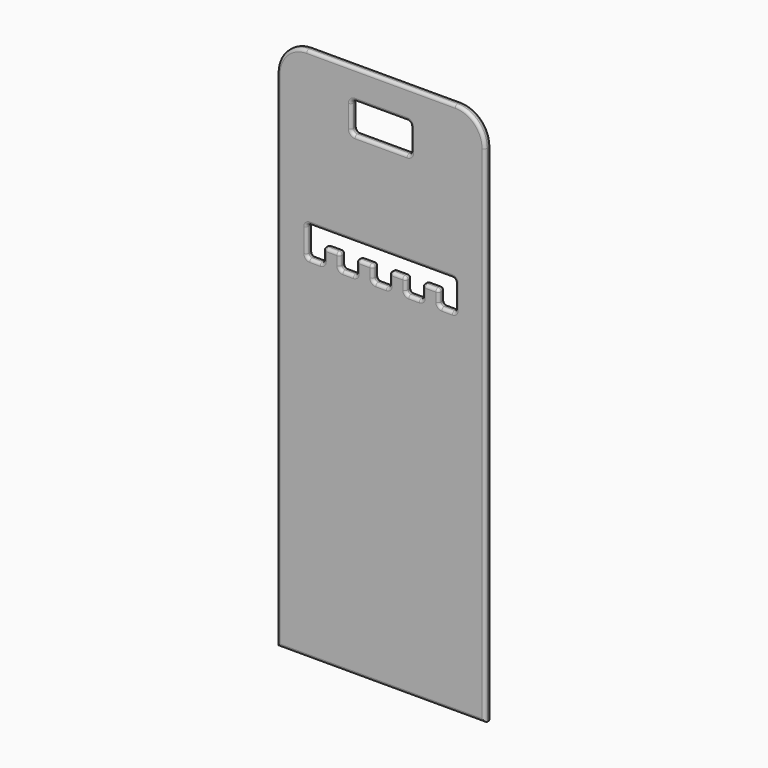
from build123d import *

# Parameters (mm, degrees)
F1_DEPTH = 12.7
F3_DEPTH = 25.4
F4_R     = 5.08
F5_R     = 5.08
F7_DEPTH = 25.4
F8_F1_R  = 5.08
F8_F2_R  = 5.08


with BuildPart() as f1:
    # F0 (on Front) → F1 (new body)
    with BuildSketch(Plane.XZ):
        with BuildLine():
            ThreePointArc((177.8, 406.4), (162.9210244843, 442.3210244843), (127, 457.2))
            Line((127, 457.2), (-127, 457.2))
            ThreePointArc((-127, 457.2), (-162.9210244843, 442.3210244843), (-177.8, 406.4))
            Line((-177.8, 406.4), (-177.8, -457.2))
            Line((-177.8, -457.2), (177.8, -457.2))
            Line((177.8, -457.2), (177.8, 406.4))
        make_face()
    extrude(amount=F1_DEPTH)

    # F2 (on face) → F3 (cut)
    with BuildSketch(Plane.XZ.offset(12.7)):
        with BuildLine():
            Line((44.45, 406.4), (0, 406.4))
            Line((0, 406.4), (-44.45, 406.4))
            ThreePointArc((-44.45, 406.4), (-48.9401280605, 404.5401280605), (-50.8, 400.05))
            Line((-50.8, 400.05), (-50.8, 361.95))
            ThreePointArc((-50.8, 361.95), (-48.9401280605, 357.4598719395), (-44.45, 355.6))
            Line((-44.45, 355.6), (44.45, 355.6))
            ThreePointArc((44.45, 355.6), (48.9401280605, 357.4598719395), (50.8, 361.95))
            Line((50.8, 361.95), (50.8, 400.05))
            ThreePointArc((50.8, 400.05), (48.9401280605, 404.5401280605), (44.45, 406.4))
        make_face()
    extrude(amount=-F3_DEPTH, mode=Mode.SUBTRACT)

    # F4
    f4_edges = [f1.edges().sort_by_distance(p)[0] for p in [
        (162.921024, -12.7, 442.321024),
        (177.8, -12.7, -25.4),
        (0, -12.7, 457.2),
        (0, -12.7, -457.2),
        (-162.921024, -12.7, 442.321024),
        (-177.8, -12.7, -25.4),
        (-48.940128, -12.7, 404.540128),
        (-50.8, -12.7, 381),
        (-48.940128, -12.7, 357.459872),
        (0, -12.7, 355.6),
        (48.940128, -12.7, 357.459872),
        (50.8, -12.7, 381),
        (48.940128, -12.7, 404.540128),
        (0, -12.7, 406.4),
    ]]
    fillet(f4_edges, radius=F4_R)

    # F5
    f5_edges = [f1.edges().sort_by_distance(p)[0] for p in [
        (162.921024, 0, 442.321024),
        (177.8, 0, -25.4),
        (0, 0, 457.2),
        (0, 0, -457.2),
        (-162.921024, 0, 442.321024),
        (-177.8, 0, -25.4),
        (0, 0, 406.4),
        (-48.940128, 0, 404.540128),
        (-50.8, 0, 381),
        (-48.940128, 0, 357.459872),
        (0, 0, 355.6),
        (48.940128, 0, 357.459872),
        (50.8, 0, 381),
        (48.940128, 0, 404.540128),
    ]]
    fillet(f5_edges, radius=F5_R)

    # F6 (on face) → F7 (cut)
    with BuildSketch(Plane.XZ.offset(12.7)):
        Polygon((127, 194.945), (0, 194.945), (-127, 194.945), (-127, 144.145), (-98.7777777778, 144.145), (-98.7777777778, 169.545), (-70.5555555556, 169.545), (-70.5555555556, 144.145), (-42.3333333333, 144.145), (-42.3333333333, 169.545), (-14.1111111111, 169.545), (-14.1111111111, 144.145), (14.1111110829, 144.145), (14.1111110829, 169.545), (42.3333333048, 169.545), (42.3333333048, 144.145), (70.5555555242, 144.145), (70.5555555242, 169.545), (98.7777777436, 169.545), (98.7777777436, 144.145), (127, 144.145), align=None)
    extrude(amount=-F7_DEPTH, mode=Mode.SUBTRACT)

    # F8: fillet of radius 5.08 on 52 edges, made by hand

    # F8_f1
    f8_f1_edges = [f1.edges().sort_by_distance(p)[0] for p in [
        (-127, -6.35, 194.945),
        (-127, -6.35, 144.145),
        (98.7777777436, -6.35, 144.145),
        (70.5555555242, -6.35, 144.145),
        (-98.7777777778, -6.35, 144.145),
        (14.1111110829, -6.35, 144.145),
        (42.3333333048, -6.35, 144.145),
        (-14.1111111111, -6.35, 144.145),
        (127, -6.35, 144.145),
        (127, -6.35, 194.945),
        (-70.5555555556, -6.35, 144.145),
        (-42.3333333333, -6.35, 144.145),
    ]]
    fillet(f8_f1_edges, radius=F8_F1_R)

    # F8_f2
    f8_f2_edges = [f1.edges().sort_by_distance(p)[0] for p in [
        (-98.7777777778, -12.7, 159.385),
        (-84.6666666667, -12.7, 169.545),
        (-70.5555555556, -12.7, 159.385),
        (-42.3333333333, -12.7, 159.385),
        (-28.2222222222, -12.7, 169.545),
        (-14.1111111111, -12.7, 159.385),
        (14.1111110829, -12.7, 159.385),
        (28.2222221938, -12.7, 169.545),
        (-42.3333333333, -6.35, 169.545),
        (98.7777777436, -6.35, 169.545),
        (70.5555555242, -6.35, 169.545),
        (84.6666666339, -12.7, 169.545),
        (70.5555555242, -12.7, 159.385),
        (-98.7777777778, 0, 159.385),
        (-70.5555555556, 0, 159.385),
        (-42.3333333333, 0, 159.385),
        (42.3333333048, -12.7, 159.385),
        (-28.2222222222, 0, 169.545),
        (14.1111110829, 0, 159.385),
        (-14.1111111111, -6.35, 169.545),
        (-98.7777777778, -6.35, 169.545),
        (-70.5555555556, -6.35, 169.545),
        (14.1111110829, -6.35, 169.545),
        (84.6666666339, 0, 169.545),
        (42.3333333048, -6.35, 169.545),
        (70.5555555242, 0, 159.385),
        (-84.6666666667, 0, 169.545),
        (-14.1111111111, 0, 159.385),
        (28.2222221938, 0, 169.545),
        (42.3333333048, 0, 159.385),
        (43.8212308564, 0, 145.6328975516),
        (-12.6232135596, 0, 145.6328975516),
        (69.0676579726, 0, 145.6328975516),
        (12.6232135313, 0, 145.6328975516),
        (43.8212308564, -12.7, 145.6328975516),
        (-43.8212308849, 0, 145.6328975516),
        (-69.067658004, 0, 145.6328975516),
        (-100.2656753294, 0, 145.6328975516),
        (69.0676579726, -12.7, 145.6328975516),
        (12.6232135313, -12.7, 145.6328975516),
        (-12.6232135596, -12.7, 145.6328975516),
        (-43.8212308849, -12.7, 145.6328975516),
        (-69.067658004, -12.7, 145.6328975516),
        (-100.2656753294, -12.7, 145.6328975516),
    ]]
    fillet(f8_f2_edges, radius=F8_F2_R)


solid = f1.part
